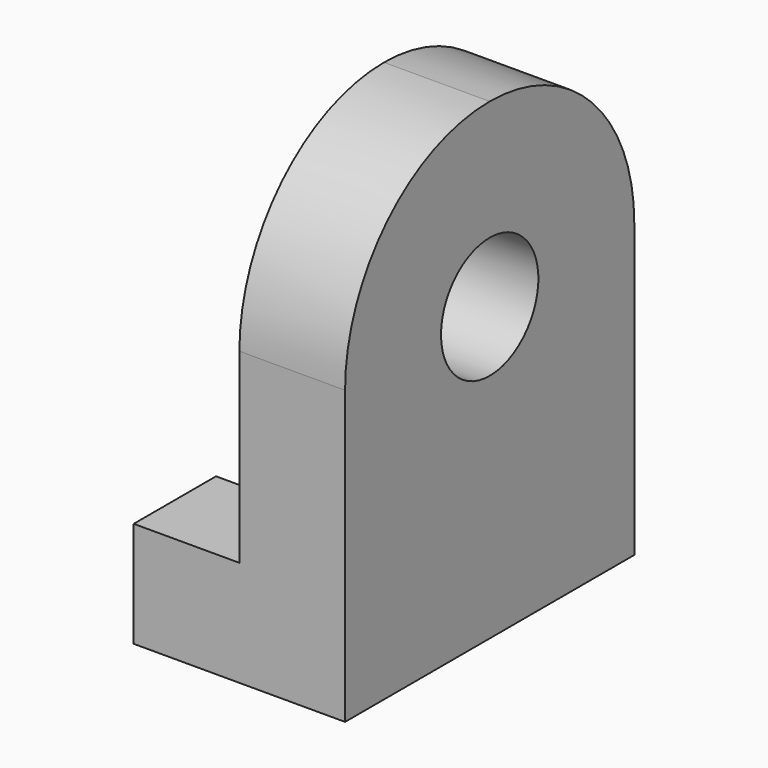
from build123d import *

# Parameters (mm, degrees)
F1_DEPTH = 66.04
F2_R     = 33.01999
F4_W     = 9.652
F4_H     = 28.448
F5_DEPTH = 30.226
F3_R     = 11.1125
F6_DEPTH = 63.246


# Not quite as in the source:
# - a fillet or chamfer is up to 0.001 mm smaller than in the source, because OpenCascade refuses the exact size


with BuildPart() as f1:
    # F0 (on Front) → F1 (new body)
    with BuildSketch(Plane.XZ):
        Polygon((0, 19.304), (0, 0), (38.608, 0), (38.608, 86.36), (19.304, 86.36), (19.304, 19.304), align=None)
    extrude(amount=F1_DEPTH)

    # F2 (radius 33.02 in the source; OpenCascade refuses exactly that, so slightly less here)
    f2_edges = [f1.edges().sort_by_distance(p)[0] for p in [
        (28.956, -66.04, 86.36),
        (28.956, 0, 86.36),
    ]]
    fillet(f2_edges, radius=F2_R)

    # F4 (on face) → F5 (cut)
    with BuildSketch(Plane.XY.offset(19.304)):
        with Locations((4.826, -33.02)):
            Rectangle(F4_W, F4_H)
    extrude(amount=-F5_DEPTH, mode=Mode.SUBTRACT)

    # F3 (on face) → F6 (cut)
    with BuildSketch(Plane(origin=(19.304, 0, 0), x_dir=(0, -1, 0), z_dir=(-1, 0, 0))):
        with Locations((33.02, 53.34)):
            Circle(F3_R)
    extrude(amount=-F6_DEPTH, mode=Mode.SUBTRACT)


solid = f1.part
